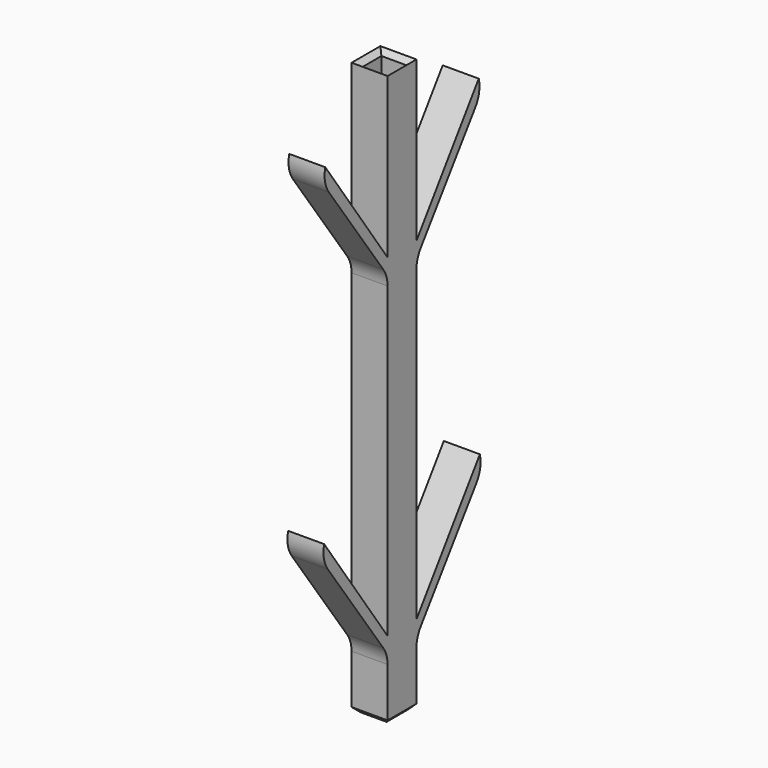
from build123d import *

# Parameters (mm, degrees)
F0_W         = 6.35
F0_H         = 6.35
F0_W_2       = 4.572
F0_H_2       = 4.572
F1_DEPTH     = 50.8
F3_T1_DEPTH  = 4.572
F3_T3_DEPTH  = 4.572
F3_T9_DEPTH  = 7.8380373947
F3_T15_DEPTH = 7.8380373947
F3_T24_DEPTH = 7.8380373947
F3_T30_DEPTH = 7.8380373947
F3_T39_DEPTH = 7.8380373947
F3_T45_DEPTH = 7.8380373947
F3_T54_DEPTH = 7.8380373947
F3_T60_DEPTH = 7.8380373947
F4_T1_DEPTH  = 12.8820747894
F4_T3_DEPTH  = 12.8820747894
F5_DEPTH     = 3.175
F6_T1_DEPTH  = 6.35
F6_T3_DEPTH  = 6.35
F6_T5_DEPTH  = 6.35
F6_T7_DEPTH  = 6.35
F6_T9_DEPTH  = 32.1381754825
F6_T11_DEPTH = 32.1381754825
F6_T13_DEPTH = 32.1381754825
F6_T15_DEPTH = 32.1381754825


# Not quite as in the source:
# - a fillet or chamfer that OpenCascade refuses, or shapes differently, is made with other operations: its cross-section is extruded or revolved along the edge and cut away or added


with BuildPart() as f1:
    # F0 (on Top) → F1 (new body, symmetric)
    with BuildSketch(Plane.XY):
        Rectangle(F0_W, F0_H)
        Rectangle(F0_W_2, F0_H_2, mode=Mode.SUBTRACT)
    extrude(amount=F1_DEPTH, both=True)

    # F3: chamfer of 1.27 on 4 edges, made by hand

    # F3_s2 → F3_t1 (cut)
    with BuildSketch(Plane.YZ.offset(-2.286)):
        Polygon((3.556, 50.8), (2.286, 49.53), (2.286, 50.8), align=None)
        Polygon((-3.556, 50.8), (-2.286, 49.53), (-2.286, 50.8), align=None)
    extrude(amount=F3_T1_DEPTH, mode=Mode.SUBTRACT)

    # F3_s4 → F3_t3 (cut)
    with BuildSketch(Plane.XZ.offset(-2.286)):
        Polygon((-3.556, 50.8), (-2.286, 49.53), (-2.286, 50.8), align=None)
        Polygon((3.556, 50.8), (2.286, 49.53), (2.286, 50.8), align=None)
    extrude(amount=F3_T3_DEPTH, mode=Mode.SUBTRACT)


with BuildPart() as f3_tool7:
    # F3_s8 → F3_t9 (new body)
    with BuildSketch(Plane.YZ.offset(-5.5520373947)):
        Polygon((3.556, 50.8), (2.286, 49.53), (2.286, 50.8), align=None)
    extrude(amount=F3_T9_DEPTH)

    split(bisect_by=Plane.YZ.offset(-3.175), keep=Keep.TOP)

    split(bisect_by=Plane.YZ.offset(-2.286), keep=Keep.BOTTOM)

    split(bisect_by=Plane.XZ.offset(-3.175), keep=Keep.TOP)


with BuildPart() as f3_tool13:
    # F3_s14 → F3_t15 (new body)
    with BuildSketch(Plane.XZ.offset(2.286)):
        Polygon((-3.556, 50.8), (-2.286, 49.53), (-2.286, 50.8), align=None)
    extrude(amount=-F3_T15_DEPTH)

    split(bisect_by=Plane.YZ.offset(-3.175), keep=Keep.TOP)

    split(bisect_by=Plane.XZ.offset(-2.286), keep=Keep.BOTTOM)

    split(bisect_by=Plane.XZ.offset(-3.175), keep=Keep.TOP)


with BuildPart() as f3_tool7_1:
    add(f3_tool7.part)

    # F3_t19: intersect F3_tool13
    add(f3_tool13.part, mode=Mode.INTERSECT)


with BuildPart() as f1_1:
    add(f1.part)

    # F3_t5: cut F3_tool7
    add(f3_tool7_1.part, mode=Mode.SUBTRACT)


with BuildPart() as f3_tool22:
    # F3_s23 → F3_t24 (new body)
    with BuildSketch(Plane.YZ.offset(-2.286)):
        Polygon((3.556, 50.8), (2.286, 49.53), (2.286, 50.8), align=None)
    extrude(amount=F3_T24_DEPTH)

    split(bisect_by=Plane.YZ.offset(3.175), keep=Keep.BOTTOM)

    split(bisect_by=Plane.YZ.offset(2.286), keep=Keep.TOP)

    split(bisect_by=Plane.XZ.offset(-3.175), keep=Keep.TOP)


with BuildPart() as f3_tool28:
    # F3_s29 → F3_t30 (new body)
    with BuildSketch(Plane.XZ.offset(-5.5520373947)):
        Polygon((3.556, 50.8), (2.286, 49.53), (2.286, 50.8), align=None)
    extrude(amount=F3_T30_DEPTH)

    split(bisect_by=Plane.YZ.offset(3.175), keep=Keep.BOTTOM)

    split(bisect_by=Plane.XZ.offset(-2.286), keep=Keep.BOTTOM)

    split(bisect_by=Plane.XZ.offset(-3.175), keep=Keep.TOP)


with BuildPart() as f3_tool22_1:
    add(f3_tool22.part)

    # F3_t34: intersect F3_tool28
    add(f3_tool28.part, mode=Mode.INTERSECT)


with BuildPart() as f1_2:
    add(f1_1.part)

    # F3_t20: cut F3_tool22
    add(f3_tool22_1.part, mode=Mode.SUBTRACT)


with BuildPart() as f3_tool37:
    # F3_s38 → F3_t39 (new body)
    with BuildSketch(Plane.YZ.offset(2.286)):
        Polygon((-3.556, 50.8), (-2.286, 49.53), (-2.286, 50.8), align=None)
    extrude(amount=-F3_T39_DEPTH)

    split(bisect_by=Plane.XZ.offset(3.175), keep=Keep.BOTTOM)

    split(bisect_by=Plane.YZ.offset(-3.175), keep=Keep.TOP)

    split(bisect_by=Plane.YZ.offset(-2.286), keep=Keep.BOTTOM)


with BuildPart() as f3_tool43:
    # F3_s44 → F3_t45 (new body)
    with BuildSketch(Plane.XZ.offset(5.5520373947)):
        Polygon((-3.556, 50.8), (-2.286, 49.53), (-2.286, 50.8), align=None)
    extrude(amount=-F3_T45_DEPTH)

    split(bisect_by=Plane.XZ.offset(3.175), keep=Keep.BOTTOM)

    split(bisect_by=Plane.YZ.offset(-3.175), keep=Keep.TOP)

    split(bisect_by=Plane.XZ.offset(2.286), keep=Keep.TOP)


with BuildPart() as f3_tool37_1:
    add(f3_tool37.part)

    # F3_t49: intersect F3_tool43
    add(f3_tool43.part, mode=Mode.INTERSECT)


with BuildPart() as f1_3:
    add(f1_2.part)

    # F3_t35: cut F3_tool37
    add(f3_tool37_1.part, mode=Mode.SUBTRACT)


with BuildPart() as f3_tool52:
    # F3_s53 → F3_t54 (new body)
    with BuildSketch(Plane.XZ.offset(-2.286)):
        Polygon((3.556, 50.8), (2.286, 49.53), (2.286, 50.8), align=None)
    extrude(amount=F3_T54_DEPTH)

    split(bisect_by=Plane.YZ.offset(3.175), keep=Keep.BOTTOM)

    split(bisect_by=Plane.XZ.offset(3.175), keep=Keep.BOTTOM)

    split(bisect_by=Plane.XZ.offset(2.286), keep=Keep.TOP)


with BuildPart() as f3_tool58:
    # F3_s59 → F3_t60 (new body)
    with BuildSketch(Plane.YZ.offset(5.5520373947)):
        Polygon((-3.556, 50.8), (-2.286, 49.53), (-2.286, 50.8), align=None)
    extrude(amount=-F3_T60_DEPTH)

    split(bisect_by=Plane.YZ.offset(3.175), keep=Keep.BOTTOM)

    split(bisect_by=Plane.XZ.offset(3.175), keep=Keep.BOTTOM)

    split(bisect_by=Plane.YZ.offset(2.286), keep=Keep.TOP)


with BuildPart() as f3_tool52_1:
    add(f3_tool52.part)

    # F3_t64: intersect F3_tool58
    add(f3_tool58.part, mode=Mode.INTERSECT)


with BuildPart() as f1_4:
    add(f1_3.part)

    # F3_t50: cut F3_tool52
    add(f3_tool52_1.part, mode=Mode.SUBTRACT)

    # F4: chamfer of 1.27 on 4 edges, made by hand

    # F4_s2 → F4_t1 (cut)
    with BuildSketch(Plane.XZ.offset(-6.4410373947)):
        Polygon((3.175, -49.53), (1.905, -50.8), (3.175, -50.8), align=None)
        Polygon((-3.175, -49.53), (-1.905, -50.8), (-3.175, -50.8), align=None)
    extrude(amount=F4_T1_DEPTH, mode=Mode.SUBTRACT)

    # F4_s4 → F4_t3 (cut)
    with BuildSketch(Plane.YZ.offset(-6.4410373947)):
        Polygon((-1.905, -50.8), (-3.175, -49.53), (-3.175, -50.8), align=None)
        Polygon((3.175, -49.53), (1.905, -50.8), (3.175, -50.8), align=None)
    extrude(amount=F4_T3_DEPTH, mode=Mode.SUBTRACT)

    # F2 (on Right) → F5 (join, symmetric)
    with BuildSketch(Plane.YZ):
        Polygon((-19.1053829622, 41.8550837785), (-2.5904842187, 18.636116758), (-2.3452136666, 21.0888255388), (-16.897945432, 41.8550837785), align=None)
        Polygon((-19.3506535143, -16.5116898715), (-2.8357547708, -39.7306568921), (-2.5904842187, -37.2779481113), (-17.1432159841, -16.5116898715), align=None)
        Polygon((2.5904842187, 18.636116758), (19.1053829622, 41.8550837785), (16.897945432, 41.8550837785), (2.3452136666, 21.0888255388), align=None)
        Polygon((17.1432159841, -16.5116898715), (2.5904842187, -37.2779481113), (2.8357547708, -39.7306568921), (19.3506535143, -16.5116898715), align=None)
    extrude(amount=F5_DEPTH, both=True)

    # F6: fillet of radius 5.08 on 8 edges, made by hand

    # F6_s2 → F6_t1 (join)
    with BuildSketch(Plane.YZ.offset(-3.175)):
        with BuildLine():
            ThreePointArc((-3.175, -40.8760570484), (-3.415789898, -39.3305973794), (-4.1153329089, -37.931646008))
            Line((-4.1153329089, -37.931646008), (-3.175, -39.2536982433))
            Line((-3.175, -39.2536982433), (-3.175, -40.8760570484))
        make_face()
    extrude(amount=F6_T1_DEPTH)

    # F6_s4 → F6_t3 (join)
    with BuildSketch(Plane.YZ.offset(-3.175)):
        with BuildLine():
            ThreePointArc((-4.1153329089, 20.7799634748), (-3.415789898, 19.3810121034), (-3.175, 17.8355524344))
            Line((-3.175, 17.8355524344), (-3.175, 19.4579112395))
            Line((-3.175, 19.4579112395), (-4.1153329089, 20.7799634748))
        make_face()
    extrude(amount=F6_T3_DEPTH)

    # F6_s6 → F6_t5 (join)
    with BuildSketch(Plane.YZ.offset(-3.175)):
        with BuildLine():
            ThreePointArc((3.175, 17.8355524344), (3.415789898, 19.3810121034), (4.1153329089, 20.7799634748))
            Line((4.1153329089, 20.7799634748), (3.175, 19.4579112395))
            Line((3.175, 19.4579112395), (3.175, 17.8355524344))
        make_face()
    extrude(amount=F6_T5_DEPTH)

    # F6_s8 → F6_t7 (join)
    with BuildSketch(Plane.YZ.offset(-3.175)):
        with BuildLine():
            ThreePointArc((3.175, -40.8760570484), (3.415789898, -39.3305973794), (4.1153329089, -37.931646008))
            Line((4.1153329089, -37.931646008), (3.175, -39.2536982433))
            Line((3.175, -39.2536982433), (3.175, -40.8760570484))
        make_face()
    extrude(amount=F6_T7_DEPTH)

    # F6_s10 → F6_t9 (cut)
    with BuildSketch(Plane.YZ.offset(-16.0690877412)):
        with BuildLine():
            ThreePointArc((-17.1432159841, -16.5116898715), (-17.2158715108, -18.6994178747), (-16.3612445142, -20.7146214221))
            Line((-16.3612445142, -20.7146214221), (-19.3506535143, -16.5116898715))
            Line((-19.3506535143, -16.5116898715), (-17.1432159841, -16.5116898715))
        make_face()
    extrude(amount=F6_T9_DEPTH, mode=Mode.SUBTRACT)

    # F6_s12 → F6_t11 (cut)
    with BuildSketch(Plane.YZ.offset(-16.0690877412)):
        with BuildLine():
            ThreePointArc((-16.1159739621, 37.6521522279), (-16.9706009587, 39.6673557754), (-16.897945432, 41.8550837785))
            Line((-16.897945432, 41.8550837785), (-19.1053829622, 41.8550837785))
            Line((-19.1053829622, 41.8550837785), (-16.1159739621, 37.6521522279))
        make_face()
    extrude(amount=F6_T11_DEPTH, mode=Mode.SUBTRACT)

    # F6_s14 → F6_t13 (cut)
    with BuildSketch(Plane.YZ.offset(-16.0690877412)):
        with BuildLine():
            ThreePointArc((16.897945432, 41.8550837785), (16.9706009587, 39.6673557754), (16.1159739621, 37.6521522279))
            Line((16.1159739621, 37.6521522279), (19.1053829622, 41.8550837785))
            Line((19.1053829622, 41.8550837785), (16.897945432, 41.8550837785))
        make_face()
    extrude(amount=F6_T13_DEPTH, mode=Mode.SUBTRACT)

    # F6_s16 → F6_t15 (cut)
    with BuildSketch(Plane.YZ.offset(-16.0690877412)):
        with BuildLine():
            ThreePointArc((17.1432159841, -16.5116898715), (17.2158715108, -18.6994178747), (16.3612445142, -20.7146214221))
            Line((16.3612445142, -20.7146214221), (19.3506535143, -16.5116898715))
            Line((19.3506535143, -16.5116898715), (17.1432159841, -16.5116898715))
        make_face()
    extrude(amount=F6_T15_DEPTH, mode=Mode.SUBTRACT)


solid = f1_4.part
